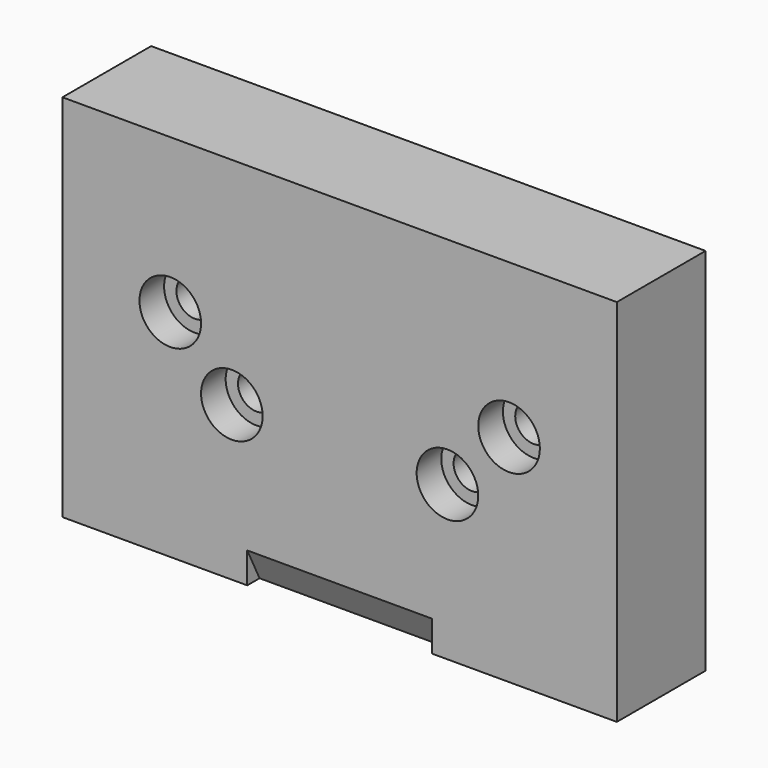
from build123d import *

# Parameters (mm, degrees)
F0_W           = 90
F0_H           = 60
F1_DEPTH       = 18
F3_D           = 6
F3_CBORE_D     = 10
F3_CBORE_DEPTH = 5
F7_DEPTH       = 30


with BuildPart() as f1:
    # F0 (on Front) → F1 (new body)
    with BuildSketch(Plane.XZ):
        with Locations((0, 30)):
            Rectangle(F0_W, F0_H)
    extrude(amount=F1_DEPTH)

    # F3 (through all)
    with Locations(Plane.XZ.offset(18)):
        with Locations((-27.5, 35), (-17.5, 25), (17.5, 25), (27.5, 35)):
            CounterBoreHole(F3_D / 2, F3_CBORE_D / 2, F3_CBORE_DEPTH)

    # F6 (on offset) → F7 (cut, through all)
    with BuildSketch(Plane(origin=(-15, 0, 0), x_dir=(0, -1, 0), z_dir=(-1, 0, 0))):
        Polygon((15.5, 0), (18, 0), (18, 5), align=None)
    extrude(amount=-F7_DEPTH, mode=Mode.SUBTRACT)


solid = f1.part
